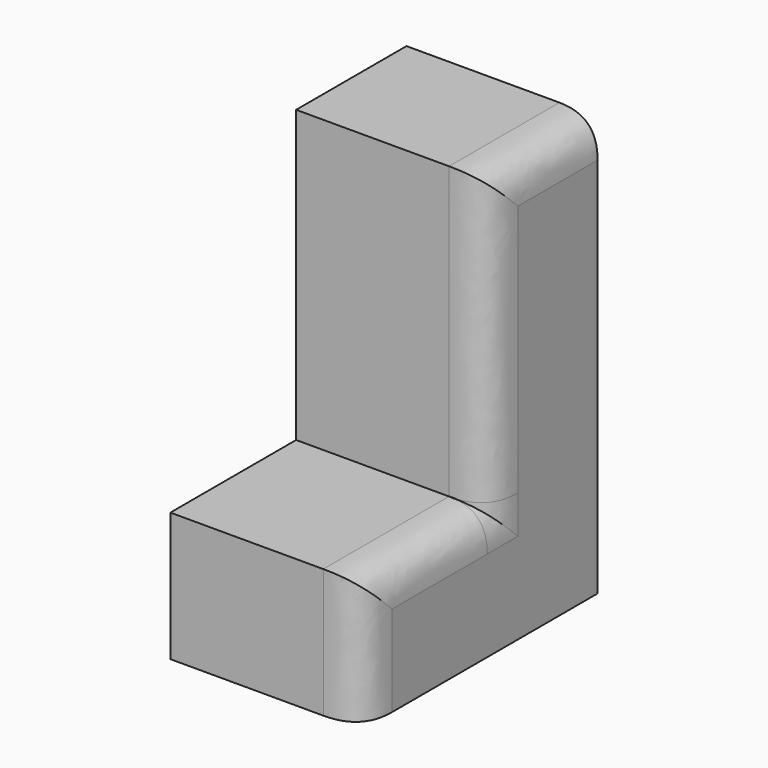
from build123d import *

# Parameters (mm, degrees)
F1_DEPTH     = 25
F2_T1_DEPTH  = 50.5172412843
F2_T3_DEPTH  = 43.0387943983
F2_T5_DEPTH  = 33.0603428185
F2_T7_DEPTH  = 41.8750006706
F2_T13_DEPTH = 63.0172412843
F2_T17_DEPTH = 45.5603428185


# Not quite as in the source:
# - a fillet or chamfer that OpenCascade refuses, or shapes differently, is made with other operations: its cross-section is extruded or revolved along the edge and cut away or added


with BuildPart() as f1:
    # F0 (on Right) → F1 (new body)
    with BuildSketch(Plane.YZ):
        Polygon((-38.5991372168, 16.8750006706), (-38.5991372168, 0), (0, 0), (0, 54.8922419548), (-18.0387943983, 54.8922419548), (-18.0387943983, 16.8750006706), align=None)
    extrude(amount=F1_DEPTH)

    # F2: fillet of radius 5 on 4 edges, made by hand

    # F2_s2 → F2_t1 (cut)
    with BuildSketch(Plane.XY.offset(16.8750006706)):
        with BuildLine():
            add(Edge.make_bspline(
                [(20, -18.0387943983), (25, -18.0387943983), (25, -13.0387943983)],
                knots=[0, 0, 0, 1, 1, 1], degree=2, weights=[1, 1, 1]))
            Line((25, -13.0387943983), (25, -18.0387943983))
            Line((25, -18.0387943983), (20, -18.0387943983))
        make_face()
    extrude(amount=F2_T1_DEPTH, mode=Mode.SUBTRACT)

    # F2_s4 → F2_t3 (cut)
    with BuildSketch(Plane.XZ.offset(-12.5)):
        with BuildLine():
            add(Edge.make_bspline(
                [(20, 54.8922419548), (25, 54.8922419548), (25, 49.8922419548)],
                knots=[0, 0, 0, 1, 1, 1], degree=2, weights=[1, 1, 1]))
            Line((25, 49.8922419548), (25, 54.8922419548))
            Line((25, 54.8922419548), (20, 54.8922419548))
        make_face()
    extrude(amount=F2_T3_DEPTH, mode=Mode.SUBTRACT)

    # F2_s6 → F2_t5 (cut)
    with BuildSketch(Plane.XZ.offset(18.0387943983)):
        with BuildLine():
            add(Edge.make_bspline(
                [(20, 16.8750006706), (25, 16.8750006706), (25, 11.8750006706)],
                knots=[0, 0, 0, 1, 1, 1], degree=2, weights=[1, 1, 1]))
            Line((25, 11.8750006706), (25, 16.8750006706))
            Line((25, 16.8750006706), (20, 16.8750006706))
        make_face()
    extrude(amount=F2_T5_DEPTH, mode=Mode.SUBTRACT)

    # F2_s8 → F2_t7 (cut)
    with BuildSketch(Plane.XY.offset(-12.5)):
        with BuildLine():
            add(Edge.make_bspline(
                [(20, -38.5991372168), (25, -38.5991372168), (25, -33.5991372168)],
                knots=[0, 0, 0, 1, 1, 1], degree=2, weights=[1, 1, 1]))
            Line((25, -33.5991372168), (25, -38.5991372168))
            Line((25, -38.5991372168), (20, -38.5991372168))
        make_face()
    extrude(amount=F2_T7_DEPTH, mode=Mode.SUBTRACT)


with BuildPart() as f2_tool11:
    # F2_s12 → F2_t13 (new body)
    with BuildSketch(Plane.XY.offset(67.3922419548)):
        with BuildLine():
            add(Edge.make_bspline(
                [(20, -18.0387943983), (25, -18.0387943983), (25, -13.0387943983)],
                knots=[0, 0, 0, 1, 1, 1], degree=2, weights=[1, 1, 1]))
            Line((25, -13.0387943983), (25, -18.0387943983))
            Line((25, -18.0387943983), (20, -18.0387943983))
        make_face()
    extrude(amount=-F2_T13_DEPTH)

    split(bisect_by=Plane.XY.offset(16.8750006706), keep=Keep.BOTTOM)


with BuildPart() as f2_tool15:
    # F2_s16 → F2_t17 (new body)
    with BuildSketch(Plane.XZ.offset(5.5387943983)):
        with BuildLine():
            add(Edge.make_bspline(
                [(20, 16.8750006706), (25, 16.8750006706), (25, 11.8750006706)],
                knots=[0, 0, 0, 1, 1, 1], degree=2, weights=[1, 1, 1]))
            Line((25, 11.8750006706), (25, 16.8750006706))
            Line((25, 16.8750006706), (20, 16.8750006706))
        make_face()
    extrude(amount=F2_T17_DEPTH)

    split(bisect_by=Plane.XZ.offset(18.0387943983), keep=Keep.BOTTOM)


with BuildPart() as f2_tool11_1:
    add(f2_tool11.part)

    # F2_t19: intersect F2_tool15
    add(f2_tool15.part, mode=Mode.INTERSECT)


with BuildPart() as f1_1:
    add(f1.part)

    # F2_t9: cut F2_tool11
    add(f2_tool11_1.part, mode=Mode.SUBTRACT)


solid = f1_1.part
